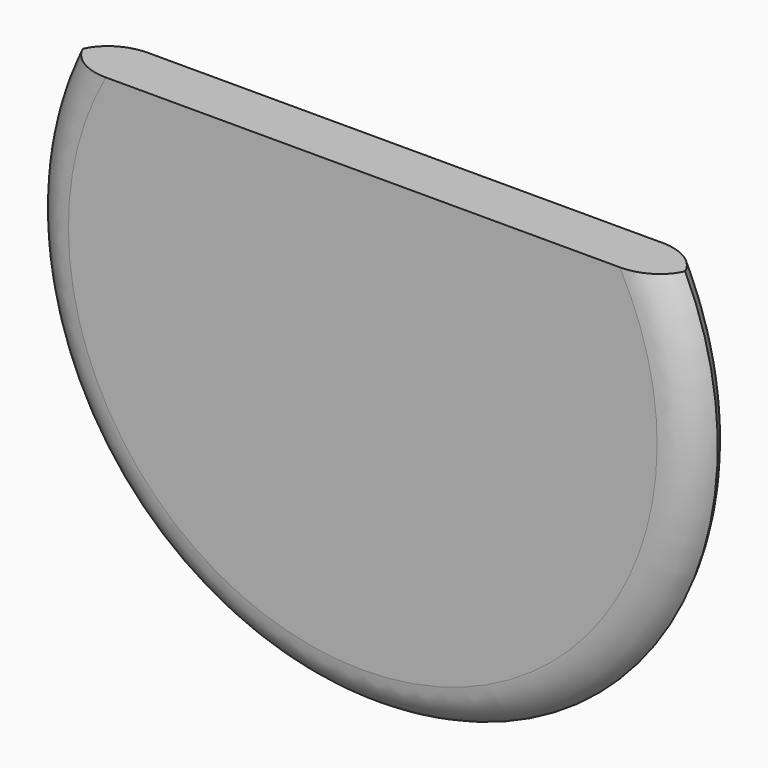
from build123d import *

# Parameters (mm, degrees)
F1_DEPTH    = 6.35
F2_T2_ANGLE = 266.7511769691
F2_T4_ANGLE = 266.7511769691


# Not quite as in the source:
# - a fillet or chamfer that OpenCascade refuses, or shapes differently, is made with other operations: its cross-section is extruded or revolved along the edge and cut away or added


with BuildPart() as f1:
    # F0 (on Front) → F1 (new body)
    with BuildSketch(Plane.XZ):
        with BuildLine():
            Line((36.234639585, 0), (-36.6263650358, 0))
            ThreePointArc((-36.6263650358, 0), (-0.1958627254, -57.476948013), (36.234639585, 0))
        make_face()
    extrude(amount=F1_DEPTH)

    # F2: fillet of radius 5.08 on 2 edges, made by hand

    # F2_s1 → F2_t2 (revolve, cut)
    with BuildSketch(Plane(origin=(-8.6751336397, 0, -9.1815294637), x_dir=(0, 1, 0), z_dir=(0.6867778831, 0, 0.7268673464))):
        with BuildLine():
            ThreePointArc((-1.27, 28.6183114219), (-4.8621024484, 27.1304138704), (-6.35, 23.5383114219))
            Line((-6.35, 23.5383114219), (-6.35, 28.6183114219))
            Line((-6.35, 28.6183114219), (-1.27, 28.6183114219))
        make_face()
    revolve(axis=Axis((-0.1958627254, -6.35, -17.1931367499), (0, -1, 0)), revolution_arc=F2_T2_ANGLE, mode=Mode.SUBTRACT)

    # F2_s3 → F2_t4 (revolve, cut)
    with BuildSketch(Plane(origin=(-8.6751336397, 0, -9.1815294637), x_dir=(0, 1, 0), z_dir=(0.6867778831, 0, 0.7268673464))):
        with BuildLine():
            ThreePointArc((-5.08, 28.6183114219), (-1.4878975516, 27.1304138704), (0, 23.5383114219))
            Line((0, 23.5383114219), (0, 28.6183114219))
            Line((0, 28.6183114219), (-5.08, 28.6183114219))
        make_face()
    revolve(axis=Axis((-0.1958627254, 0, -17.1931367499), (0, -1, 0)), revolution_arc=F2_T4_ANGLE, mode=Mode.SUBTRACT)


solid = f1.part
